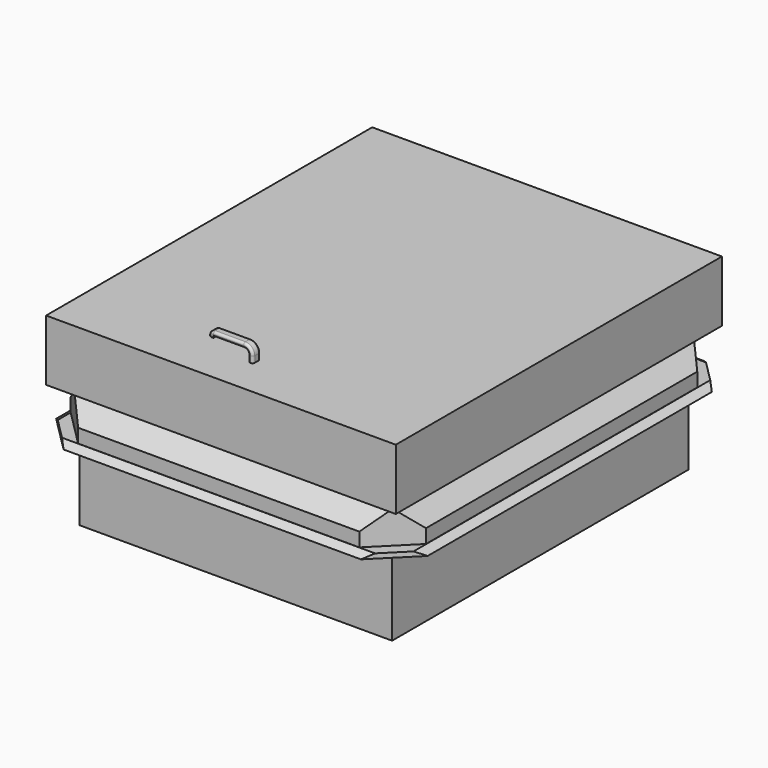
from build123d import *

# Parameters (mm, degrees)
F0_W          = 675
F0_H          = 800
F1_DEPTH      = 270
F2_W          = 755
F2_H          = 880
F3_DEPTH      = 131.76
F5_START      = -175
F4_W          = 802
F4_H          = 926.8378600104
F5_DEPTH      = 10
F6_W          = 767
F6_H          = 892
F7_DEPTH      = 70
F8_SIZE       = 80
F9_SIZE       = 39.99999
F10_SIZE2     = 9.99999
F10_SIZE      = 16.99999
F13_W         = 10
F13_H         = 20
F15_R         = 3.5
F16_T1_DEPTH  = 65
F16_T3_DEPTH  = 3.5995793343
F16_T5_DEPTH  = 13.4709453487
F16_T8_ANGLE  = 90
F16_T10_ANGLE = 90
F16_T12_ANGLE = 90
F16_T14_ANGLE = 90
F16_T16_ANGLE = 90
F16_T18_ANGLE = 90
F16_T20_ANGLE = 90
F16_T22_ANGLE = 90


# Not quite as in the source:
# - a fillet or chamfer that OpenCascade refuses, or shapes differently, is made with other operations: its cross-section is extruded or revolved along the edge and cut away or added
# - a fillet or chamfer is up to 0.001 mm smaller than in the source, because OpenCascade refuses the exact size
# - a feature names something its author has since deleted; it is built from what else it names


with BuildPart() as f1:
    # F0 (on Top) → F1 (new body)
    with BuildSketch(Plane.XY):
        Rectangle(F0_W, F0_H)
    extrude(amount=F1_DEPTH)

    # F2 (on face) → F3 (join)
    with BuildSketch(Plane.XY.offset(270)):
        Rectangle(F2_W, F2_H)
    extrude(amount=F3_DEPTH)

    # F4 (on face) → F5 (join)
    with BuildSketch(Plane(origin=(0, 0, 0), x_dir=(1, 0, 0), z_dir=(0, 0, -1)).offset(F5_START)):
        Rectangle(F4_W, F4_H)
    extrude(amount=-F5_DEPTH)

    # F6 (on face) → F7 (join)
    with BuildSketch(Plane.XY.offset(185)):
        Rectangle(F6_W, F6_H)
    extrude(amount=F7_DEPTH)

    # F8
    f8_edges = [f1.edges().sort_by_distance(p)[0] for p in [
        (383.5, 446, 220),
        (-383.5, 446, 220),
        (-383.5, -446, 220),
        (-401, 463.41893, 180),
        (-401, -463.41893, 180),
        (401, 463.41893, 180),
        (401, -463.41893, 180),
        (383.5, -446, 220),
    ]]
    chamfer(f8_edges, length=F8_SIZE)

    # F9 (size 40 in the source; OpenCascade refuses exactly that, so slightly less here)
    f9_edges = [f1.edges().sort_by_distance(p)[0] for p in [
        (383.5, 0, 255),
        (-383.5, 0, 255),
        (0, 446, 255),
        (0, -446, 255),
    ]]
    chamfer(f9_edges, length=F9_SIZE)

    # F10 (size 17 and 10 in the source; OpenCascade refuses exactly that, so slightly less here)
    f10_edges = [f1.edges().sort_by_distance(p)[0] for p in [
        (-401, 0, 185),
        (0, 463.41893, 185),
        (0, -463.41893, 185),
        (401, 0, 185),
    ]]
    chamfer(f10_edges, length=F10_SIZE, length2=F10_SIZE2)

    # F14: sweep along a path in F12
    with BuildLine(Plane.XZ.offset(350)) as f14_path:
        Line((0, 401.76), (0, 415.2309453487))
        ThreePointArc((0, 415.2309453487), (-4.3933982822, 425.8375470665), (-15, 430.2309453487))
        Line((-15, 430.2309453487), (-80, 430.2309453487))
        ThreePointArc((-80, 430.2309453487), (-83.5355339059, 428.7664792547), (-85, 425.2309453487))
        Line((-85, 425.2309453487), (-85, 421.6313660145))
    # F13 (on face) → F14 (sweep)
    with BuildSketch(Plane.XY.offset(401.76)):
        with Locations((0, -350)):
            Rectangle(F13_W, F13_H)
    sweep(path=f14_path.line)

    # F15
    f15_edges = [f1.edges().sort_by_distance(p)[0] for p in [
        (-90, -350, 421.631366),
        (-85, -360, 421.631366),
        (-80, -350, 421.631366),
        (-85, -340, 421.631366),
    ]]
    fillet(f15_edges, radius=F15_R)

    # F16: fillet of radius 5 on 16 edges, made by hand

    # F16_s2 → F16_t1 (cut)
    with BuildSketch(Plane.YZ.offset(-80)):
        with BuildLine():
            ThreePointArc((-360, 430.2309453487), (-358.5355339059, 433.7664792547), (-355, 435.2309453487))
            Line((-355, 435.2309453487), (-360, 435.2309453487))
            Line((-360, 435.2309453487), (-360, 430.2309453487))
        make_face()
        with BuildLine():
            ThreePointArc((-345, 435.2309453487), (-341.4644660941, 433.7664792547), (-340, 430.2309453487))
            Line((-340, 430.2309453487), (-340, 435.2309453487))
            Line((-340, 435.2309453487), (-345, 435.2309453487))
        make_face()
        with BuildLine():
            ThreePointArc((-360, 430.2309453487), (-358.5355339059, 426.6954114428), (-355, 425.2309453487))
            Line((-355, 425.2309453487), (-360, 425.2309453487))
            Line((-360, 425.2309453487), (-360, 430.2309453487))
        make_face()
        with BuildLine():
            ThreePointArc((-345, 425.2309453487), (-341.4644660941, 426.6954114428), (-340, 430.2309453487))
            Line((-340, 430.2309453487), (-340, 425.2309453487))
            Line((-340, 425.2309453487), (-345, 425.2309453487))
        make_face()
    extrude(amount=F16_T1_DEPTH, mode=Mode.SUBTRACT)

    # F16_s4 → F16_t3 (cut)
    with BuildSketch(Plane.XY.offset(421.6313660145)):
        with BuildLine():
            ThreePointArc((-85, -360), (-88.5355339059, -358.5355339059), (-90, -355))
            Line((-90, -355), (-90, -360))
            Line((-90, -360), (-85, -360))
        make_face()
        with BuildLine():
            ThreePointArc((-90, -345), (-88.5355339059, -341.4644660941), (-85, -340))
            Line((-85, -340), (-90, -340))
            Line((-90, -340), (-90, -345))
        make_face()
    extrude(amount=F16_T3_DEPTH, mode=Mode.SUBTRACT)

    # F16_s6 → F16_t5 (cut)
    with BuildSketch(Plane.XY.offset(401.76)):
        with BuildLine():
            ThreePointArc((0, -360), (3.5355339059, -358.5355339059), (5, -355))
            Line((5, -355), (5, -360))
            Line((5, -360), (0, -360))
        make_face()
        with BuildLine():
            ThreePointArc((0, -360), (-3.5355339059, -358.5355339059), (-5, -355))
            Line((-5, -355), (-5, -360))
            Line((-5, -360), (0, -360))
        make_face()
        with BuildLine():
            ThreePointArc((5, -345), (3.5355339059, -341.4644660941), (0, -340))
            Line((0, -340), (5, -340))
            Line((5, -340), (5, -345))
        make_face()
        with BuildLine():
            ThreePointArc((-5, -345), (-3.5355339059, -341.4644660941), (0, -340))
            Line((0, -340), (-5, -340))
            Line((-5, -340), (-5, -345))
        make_face()
    extrude(amount=F16_T5_DEPTH, mode=Mode.SUBTRACT)

    # F16_s7 → F16_t8 (revolve, cut)
    with BuildSketch(Plane.XZ.offset(345)):
        with BuildLine():
            ThreePointArc((-86.5, 421.6313660145), (-88.9748737342, 422.6564922803), (-90, 425.1313660145))
            Line((-90, 425.1313660145), (-90, 421.6313660145))
            Line((-90, 421.6313660145), (-86.5, 421.6313660145))
        make_face()
    revolve(axis=Axis((-85, -345, 421.6313660145), (0, 0, -1)), revolution_arc=F16_T8_ANGLE, mode=Mode.SUBTRACT)

    # F16_s9 → F16_t10 (revolve, cut)
    with BuildSketch(Plane.YZ.offset(-85)):
        with BuildLine():
            ThreePointArc((-356.5, 421.6313660145), (-358.9748737342, 422.6564922803), (-360, 425.1313660145))
            Line((-360, 425.1313660145), (-360, 421.6313660145))
            Line((-360, 421.6313660145), (-356.5, 421.6313660145))
        make_face()
    revolve(axis=Axis((-85, -355, 421.6313660145), (0, 0, -1)), revolution_arc=F16_T10_ANGLE, mode=Mode.SUBTRACT)

    # F16_s11 → F16_t12 (revolve, cut)
    with BuildSketch(Plane.YZ.offset(-80)):
        with BuildLine():
            ThreePointArc((-360, 430.2309453487), (-358.5355339059, 433.7664792547), (-355, 435.2309453487))
            Line((-355, 435.2309453487), (-360, 435.2309453487))
            Line((-360, 435.2309453487), (-360, 430.2309453487))
        make_face()
    revolve(axis=Axis((-80, -360, 425.2309453487), (0, -1, 0)), revolution_arc=F16_T12_ANGLE, mode=Mode.SUBTRACT)

    # F16_s13 → F16_t14 (revolve, cut)
    with BuildSketch(Plane.XY.offset(415.2309453487)):
        with BuildLine():
            ThreePointArc((0, -360), (3.5355339059, -358.5355339059), (5, -355))
            Line((5, -355), (5, -360))
            Line((5, -360), (0, -360))
        make_face()
    revolve(axis=Axis((-15, -360, 415.2309453487), (0, -1, 0)), revolution_arc=F16_T14_ANGLE, mode=Mode.SUBTRACT)

    # F16_s15 → F16_t16 (revolve, cut)
    with BuildSketch(Plane.XY.offset(415.2309453487)):
        with BuildLine():
            ThreePointArc((0, -360), (-3.5355339059, -358.5355339059), (-5, -355))
            Line((-5, -355), (-5, -360))
            Line((-5, -360), (0, -360))
        make_face()
    revolve(axis=Axis((-15, -360, 415.2309453487), (0, -1, 0)), revolution_arc=F16_T16_ANGLE, mode=Mode.SUBTRACT)

    # F16_s17 → F16_t18 (revolve, cut)
    with BuildSketch(Plane.YZ.offset(-80)):
        with BuildLine():
            ThreePointArc((-345, 435.2309453487), (-341.4644660941, 433.7664792547), (-340, 430.2309453487))
            Line((-340, 430.2309453487), (-340, 435.2309453487))
            Line((-340, 435.2309453487), (-345, 435.2309453487))
        make_face()
    revolve(axis=Axis((-80, -340, 425.2309453487), (0, -1, 0)), revolution_arc=F16_T18_ANGLE, mode=Mode.SUBTRACT)

    # F16_s19 → F16_t20 (revolve, cut)
    with BuildSketch(Plane.XY.offset(415.2309453487)):
        with BuildLine():
            ThreePointArc((5, -345), (3.5355339059, -341.4644660941), (0, -340))
            Line((0, -340), (5, -340))
            Line((5, -340), (5, -345))
        make_face()
    revolve(axis=Axis((-15, -340, 415.2309453487), (0, -1, 0)), revolution_arc=F16_T20_ANGLE, mode=Mode.SUBTRACT)

    # F16_s21 → F16_t22 (revolve, cut)
    with BuildSketch(Plane.XY.offset(415.2309453487)):
        with BuildLine():
            ThreePointArc((-5, -345), (-3.5355339059, -341.4644660941), (0, -340))
            Line((0, -340), (-5, -340))
            Line((-5, -340), (-5, -345))
        make_face()
    revolve(axis=Axis((-15, -340, 415.2309453487), (0, -1, 0)), revolution_arc=F16_T22_ANGLE, mode=Mode.SUBTRACT)


solid = f1.part
